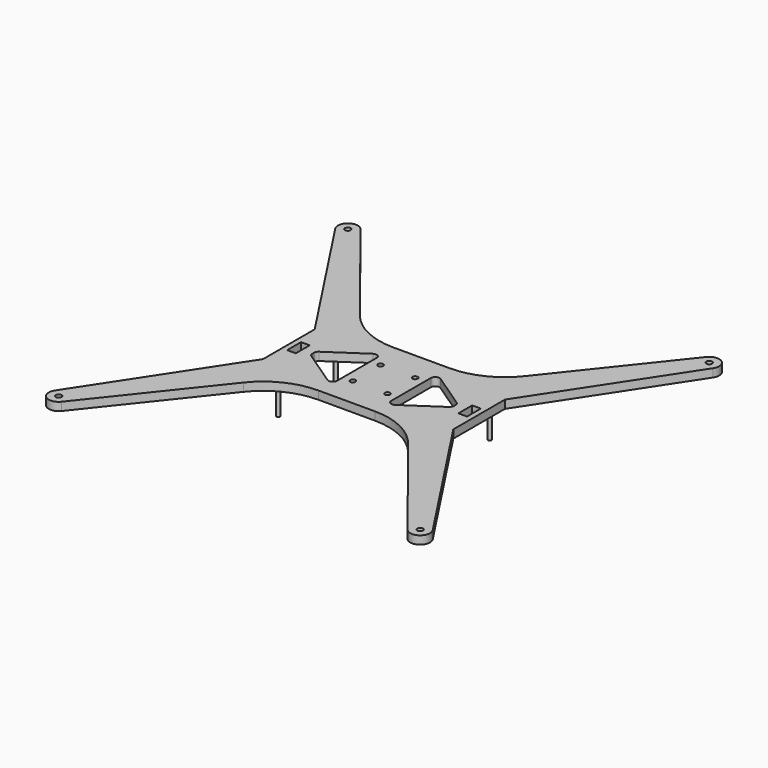
from build123d import *

# Parameters (mm, degrees)
F0_R     = 1.65
F0_R_2   = 2.55
F0_W     = 5
F0_H     = 10
F0_R_3   = 1.5
F0_R_4   = 3.555
F1_DEPTH = 4.75
F2_R     = 1
F3_DEPTH = 20
F4_R     = 3.555
F4_R_2   = 2.55
F5_DEPTH = 4.75


# Not quite as in the source:
# - ends of sketch curves that miss each other by under 0.0002 mm in the source are joined


with BuildPart() as f1:
    # F0 (on Top) → F1 (new body)
    with BuildSketch(Plane.XY):
        with BuildLine():
            Line((-47.640397, 42.115595), (-100.031737, 108.050449))
            ThreePointArc((-100.031737, 108.050449), (-107.8442155419, 109.1246397394), (-109.2715048598, 101.368896092))
            Line((-109.2715048598, 101.368896092), (-54.999977, 18.664241))
            Line((-54.999977, 18.664241), (-54.999977, -18.664242))
            Line((-54.999977, -18.664242), (-109.271505, -101.368897))
            ThreePointArc((-109.271505, -101.368897), (-107.8441644553, -109.1246766812), (-100.031658534, -108.0503513703))
            Line((-100.031658534, -108.0503513703), (-47.643302, -42.116283))
            ThreePointArc((-47.643302, -42.116283), (-33.7130803066, -30.9767526972), (-16.325566, -27))
            Line((-16.325566, -27), (16.325565, -27))
            ThreePointArc((16.325565, -27), (33.7130793066, -30.9767526972), (47.6433013924, -42.1162826882))
            Line((47.6433013924, -42.1162826882), (100.031658, -108.050351))
            ThreePointArc((100.031658, -108.050351), (107.8441644255, -109.1246767027), (109.2715050175, -101.3688963323))
            Line((109.2715050175, -101.3688963323), (54.999976, -18.664242))
            Line((54.999976, -18.664242), (54.999976, 18.664241))
            Line((54.999976, 18.664241), (109.271504, 101.368896))
            ThreePointArc((109.271504, 101.368896), (107.8442155121, 109.1246397609), (100.0317360662, 108.0504489474))
            Line((100.0317360662, 108.0504489474), (47.640396, 42.115595))
            ThreePointArc((47.640396, 42.115595), (33.7103248028, 30.9765618002), (16.323206, 27))
            Line((16.323206, 27), (-16.323206, 27))
            ThreePointArc((-16.323206, 27), (-33.710325083, 30.9765619354), (-47.640397, 42.115595))
        make_face()
        with Locations((-104.5, -104.5)):
            Circle(F0_R, mode=Mode.SUBTRACT)
        with Locations((-44.444977, -20.807752)):
            Circle(F0_R_2, mode=Mode.SUBTRACT)
        with Locations((-49.499977, 0)):
            Rectangle(F0_W, F0_H, mode=Mode.SUBTRACT)
        with BuildLine():
            Line((-19.581953, -16.373154), (-39.803759, -2.743263))
            ThreePointArc((-39.803759, -2.743263), (-40.6136447533, -1.8442487652), (-40.906473, -0.670199))
            Line((-40.906473, -0.670199), (-40.906473, 0.670176))
            ThreePointArc((-40.906473, 0.670176), (-40.6136450793, 1.8442251525), (-39.8037598701, 2.7432388072))
            Line((-39.8037598701, 2.7432388072), (-19.581955, 16.373149))
            ThreePointArc((-19.581955, 16.373149), (-17.0106188475, 16.5072580793), (-15.684668, 14.300086))
            Line((-15.684668, 14.300086), (-15.684668, -14.30009))
            ThreePointArc((-15.684668, -14.30009), (-17.0106178687, -16.5072615586), (-19.581953, -16.373154))
        make_face(mode=Mode.SUBTRACT)
        with Locations((-10, -10)):
            Circle(F0_R_3, mode=Mode.SUBTRACT)
        with Locations((104.5, -104.5)):
            Circle(F0_R, mode=Mode.SUBTRACT)
        with Locations((10, -10)):
            Circle(F0_R_3, mode=Mode.SUBTRACT)
        with Locations((44.444976, -20.807752)):
            Circle(F0_R_2, mode=Mode.SUBTRACT)
        with BuildLine():
            Line((19.581954, 16.373149), (39.803759, 2.743239))
            ThreePointArc((39.803759, 2.743239), (40.6136440793, 1.8442251525), (40.906472, 0.670176))
            Line((40.906472, 0.670176), (40.906472, -0.670199))
            ThreePointArc((40.906472, -0.670199), (40.6136437533, -1.8442487652), (39.803757719, -2.7432625831))
            Line((39.803757719, -2.7432625831), (19.581952, -16.373154))
            ThreePointArc((19.581952, -16.373154), (17.0106168687, -16.5072615586), (15.684667, -14.30009))
            Line((15.684667, -14.30009), (15.684667, 14.300086))
            ThreePointArc((15.684667, 14.300086), (17.0106178475, 16.5072580793), (19.581954, 16.373149))
        make_face(mode=Mode.SUBTRACT)
        with Locations((49.499976, 0)):
            Rectangle(F0_W, F0_H, mode=Mode.SUBTRACT)
        with Locations((-44.444977, 20.810818)):
            Circle(F0_R_4, mode=Mode.SUBTRACT)
        with Locations((-10, 10)):
            Circle(F0_R_3, mode=Mode.SUBTRACT)
        with Locations((-104.5, 104.5)):
            Circle(F0_R, mode=Mode.SUBTRACT)
        with Locations((10, 10)):
            Circle(F0_R_3, mode=Mode.SUBTRACT)
        with Locations((44.444976, 20.810818)):
            Circle(F0_R_4, mode=Mode.SUBTRACT)
        with Locations((104.5, 104.5)):
            Circle(F0_R, mode=Mode.SUBTRACT)
    extrude(amount=F1_DEPTH)



with BuildPart() as f3:
    # F2 (on Top) → F3 (new body)
    with BuildSketch(Plane.XY):
        with Locations((-44.444977, 20.810818)):
            Circle(F2_R)
    extrude(amount=-F3_DEPTH)


with BuildPart() as f3b:
    # F2 (on Top) → F3, piece 2 (new body)
    with BuildSketch(Plane.XY):
        with Locations((44.444976, 20.810818)):
            Circle(F2_R)
    extrude(amount=-F3_DEPTH)


with BuildPart() as f3c:
    # F2 (on Top) → F3, piece 3 (new body)
    with BuildSketch(Plane.XY):
        with Locations((-44.444977, -20.807752)):
            Circle(F2_R)
    extrude(amount=-F3_DEPTH)


with BuildPart() as f3d:
    # F2 (on Top) → F3, piece 4 (new body)
    with BuildSketch(Plane.XY):
        with Locations((44.444976, -20.807752)):
            Circle(F2_R)
    extrude(amount=-F3_DEPTH)


with BuildPart() as f1_1:
    add(f1.part)

    add(f3.part)  # F5 merges F3

    add(f3b.part)  # F5 merges F3b

    add(f3c.part)  # F5 merges F3c

    add(f3d.part)  # F5 merges F3d
    # F4 (on face) → F5 (join)
    with BuildSketch(Plane.XY.offset(4.75)):
        with Locations((-44.444977, 20.810818)):
            Circle(F4_R)
        with Locations((-44.444977, -20.807752)):
            Circle(F4_R_2)
        with Locations((44.444976, 20.810818)):
            Circle(F4_R)
        with Locations((44.444976, -20.807752)):
            Circle(F4_R_2)
    extrude(amount=-F5_DEPTH)


solid = f1_1.part
